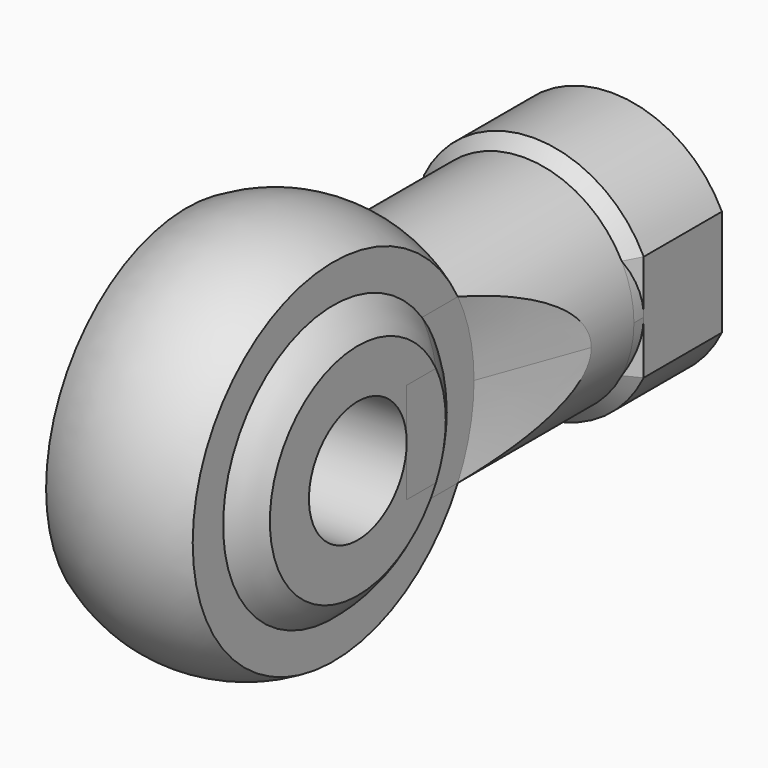
from build123d import *

# Parameters (mm, degrees)
F9_R          = 2.5
F10_DEPTH     = 15.5
F11_DEPTH     = 4.5
F12_DEPTH     = 6.5
F13_T2_ANGLE  = 157.8095212227
F13_T6_DEPTH  = 3.4652909658
F13_S7_R      = 4.5
F13_T8_DEPTH  = 3
F13_T12_DEPTH = 3.4652909658
F13_S13_R     = 4.5
F13_T14_DEPTH = 3
F13_T16_ANGLE = 157.8095212227
F13_T20_DEPTH = 3.4652909658
F13_S21_R     = 4.5
F13_T22_DEPTH = 3
F13_T26_DEPTH = 3.4652909658
F13_S27_R     = 4.5
F13_T28_DEPTH = 3


# Not quite as in the source:
# - a fillet or chamfer that OpenCascade refuses, or shapes differently, is made with other operations: its cross-section is extruded or revolved along the edge and cut away or added


with BuildPart() as f7:
    # F6 (on Top) → F7 (revolve)
    with BuildSketch(Plane.XY):
        with BuildLine():
            Line((-4, 4.5), (-4, 2.5))
            Line((-4, 2.5), (4, 2.5))
            Line((4, 2.5), (4, 4.5))
            ThreePointArc((4, 4.5), (3.5461149614, 5.1104772433), (3, 5.6400549446))
            ThreePointArc((3, 5.6400549446), (0, 6.716990566), (-3, 5.6400549446))
            ThreePointArc((-3, 5.6400549446), (-3.5461149614, 5.1104772433), (-4, 4.5))
        make_face()
        with BuildLine():
            Line((-3, 7.1961524227), (-3, 5.6400549446))
            ThreePointArc((-3, 5.6400549446), (0, 6.716990566), (3, 5.6400549446))
            Line((3, 5.6400549446), (3, 7.1961524227))
            ThreePointArc((3, 7.1961524227), (0, 8), (-3, 7.1961524227))
        make_face()
    revolve(axis=Axis((0, 0, 0), (1, 0, 0)))

    # F9 (on offset) → F10 (join)
    with BuildSketch(Plane.XZ.offset(-18)):
        with BuildLine():
            ThreePointArc((-4.5, 0), (0, -4.5), (4.5, 0))
            ThreePointArc((4.5, 0), (0, 4.5), (-4.5, 0))
        make_face()
        Circle(F9_R, mode=Mode.SUBTRACT)
        Circle(F9_R)
    extrude(amount=F10_DEPTH)

    # F9 (on offset) → F11 (join)
    with BuildSketch(Plane.XZ.offset(-18)):
        with BuildLine():
            ThreePointArc((-4.5, 0), (0, 4.5), (4.5, 0))
            Line((4.5, 0), (4.5, 2.1794494718))
            ThreePointArc((4.5, 2.1794494718), (0, 5), (-4.5, 2.1794494718))
            Line((-4.5, 2.1794494718), (-4.5, 0))
        make_face()
        with BuildLine():
            Line((4.5, -2.1794494718), (4.5, 0))
            ThreePointArc((4.5, 0), (0, -4.5), (-4.5, 0))
            Line((-4.5, 0), (-4.5, -2.1794494718))
            ThreePointArc((-4.5, -2.1794494718), (0, -5), (4.5, -2.1794494718))
        make_face()
    extrude(amount=F11_DEPTH)

    # F9 (on offset) → F12 (cut)
    with BuildSketch(Plane.XZ.offset(-18)):
        Circle(F9_R)
    extrude(amount=F12_DEPTH, mode=Mode.SUBTRACT)

    # F13: chamfer of 0.5 on 6 edges, made by hand

    # F13_s1 → F13_t2 (revolve, cut)
    with BuildSketch(Plane(origin=(0, 0, 0), x_dir=(0, 1, 0), z_dir=(0.1924404319, 0, -0.9813086569))):
        Polygon((13.5, 4.5), (14, 5), (13.5, 5), align=None)
    revolve(axis=Axis((0, 13.5, 0), (0, -1, 0)), revolution_arc=F13_T2_ANGLE, mode=Mode.SUBTRACT)


with BuildPart() as f13_tool4:
    # F13_s5 → F13_t6 (new body)
    with BuildSketch(Plane.XY):
        Polygon((4, 13.5), (4.5, 14), (4.5, 13.5), align=None)
    extrude(amount=F13_T6_DEPTH)

    # F13_s7 → F13_t8 (cut, symmetric)
    with BuildSketch(Plane.XZ.offset(-13.8)):
        Circle(F13_S7_R)
    extrude(amount=F13_T8_DEPTH, both=True, mode=Mode.SUBTRACT)


with BuildPart() as f7_1:
    add(f7.part)

    # F13_t3: cut F13_tool4
    add(f13_tool4.part, mode=Mode.SUBTRACT)


with BuildPart() as f13_tool10:
    # F13_s11 → F13_t12 (new body)
    with BuildSketch(Plane.XY.offset(3.4652909658)):
        Polygon((-4, 13.5), (-4.5, 14), (-4.5, 13.5), align=None)
    extrude(amount=-F13_T12_DEPTH)

    # F13_s13 → F13_t14 (cut, symmetric)
    with BuildSketch(Plane.XZ.offset(-13.8)):
        Circle(F13_S13_R)
    extrude(amount=F13_T14_DEPTH, both=True, mode=Mode.SUBTRACT)


with BuildPart() as f7_2:
    add(f7_1.part)

    # F13_t9: cut F13_tool10
    add(f13_tool10.part, mode=Mode.SUBTRACT)

    # F13_s15 → F13_t16 (revolve, cut)
    with BuildSketch(Plane(origin=(0, 0, 0), x_dir=(0, 1, 0), z_dir=(-0.1924404319, 0, 0.9813086569))):
        Polygon((13.5, 4.5), (14, 5), (13.5, 5), align=None)
    revolve(axis=Axis((0, 13.5, 0), (0, -1, 0)), revolution_arc=F13_T16_ANGLE, mode=Mode.SUBTRACT)


with BuildPart() as f13_tool18:
    # F13_s19 → F13_t20 (new body)
    with BuildSketch(Plane.XY.offset(-3.4652909658)):
        Polygon((4, 13.5), (4.5, 14), (4.5, 13.5), align=None)
    extrude(amount=F13_T20_DEPTH)

    # F13_s21 → F13_t22 (cut, symmetric)
    with BuildSketch(Plane.XZ.offset(-13.8)):
        Circle(F13_S21_R)
    extrude(amount=F13_T22_DEPTH, both=True, mode=Mode.SUBTRACT)


with BuildPart() as f7_3:
    add(f7_2.part)

    # F13_t17: cut F13_tool18
    add(f13_tool18.part, mode=Mode.SUBTRACT)


with BuildPart() as f13_tool24:
    # F13_s25 → F13_t26 (new body)
    with BuildSketch(Plane.XY):
        Polygon((-4, 13.5), (-4.5, 14), (-4.5, 13.5), align=None)
    extrude(amount=-F13_T26_DEPTH)

    # F13_s27 → F13_t28 (cut, symmetric)
    with BuildSketch(Plane.XZ.offset(-13.8)):
        Circle(F13_S27_R)
    extrude(amount=F13_T28_DEPTH, both=True, mode=Mode.SUBTRACT)


with BuildPart() as f7_4:
    add(f7_3.part)

    # F13_t23: cut F13_tool24
    add(f13_tool24.part, mode=Mode.SUBTRACT)

    # F6 (on Top) → F14 (revolve, cut)
    with BuildSketch(Plane.XY):
        with BuildLine():
            Line((4, 4.5), (4, 2.5))
            Line((4, 2.5), (6, 2.5))
            Line((6, 2.5), (6, 11.5))
            Line((6, 11.5), (4.566472411, 11.5))
            Line((4.566472411, 11.5), (3, 7.1961524227))
            Line((3, 7.1961524227), (3, 5.6400549446))
            ThreePointArc((3, 5.6400549446), (3.5461149614, 5.1104772433), (4, 4.5))
        make_face()
        with BuildLine():
            Line((-6, 2.5), (-4, 2.5))
            Line((-4, 2.5), (-4, 4.5))
            ThreePointArc((-4, 4.5), (-3.5461149614, 5.1104772433), (-3, 5.6400549446))
            Line((-3, 5.6400549446), (-3, 7.1961524227))
            Line((-3, 7.1961524227), (-4.566472411, 11.5))
            Line((-4.566472411, 11.5), (-6, 11.5))
            Line((-6, 11.5), (-6, 2.5))
        make_face()
    revolve(axis=Axis((0, 0, 0), (1, 0, 0)), mode=Mode.SUBTRACT)


solid = f7_4.part
